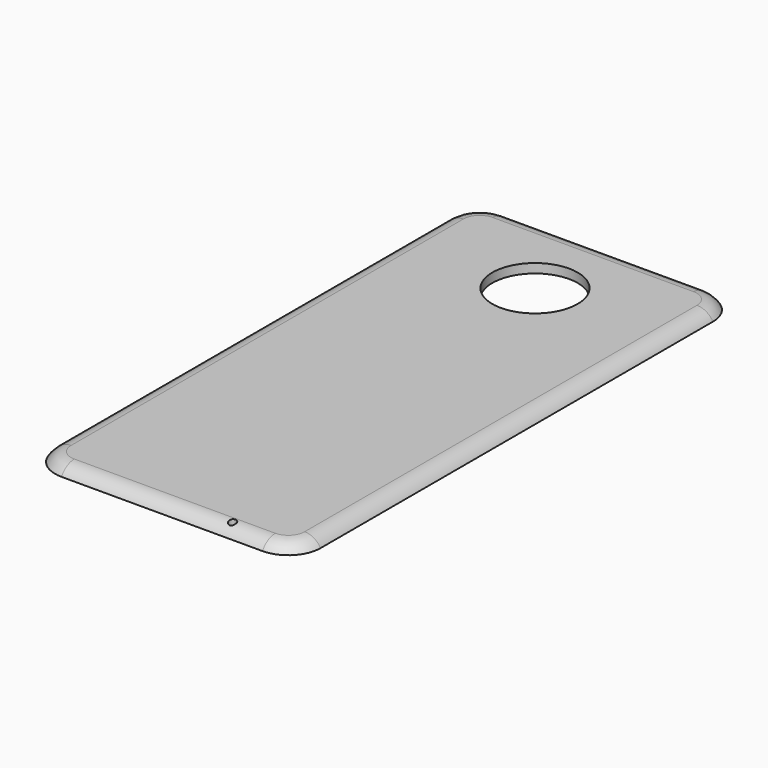
from build123d import *

# Parameters (mm, degrees)
F1_DEPTH     = 2.54
F2_R         = 11.75
F3_DEPTH     = 2.541
F4_R         = 8.89
F5_T1_DEPTH  = 135.128
F5_T3_DEPTH  = 55.372
F5_T6_ANGLE  = 90
F5_T8_ANGLE  = 90
F5_T10_ANGLE = 90
F5_T12_ANGLE = 90
F6_R         = 1
F7_DEPTH     = 2.541
F9_R         = 1.6
F8_R         = 1.6
F10_DEPTH    = 1.2
F11_R        = 2.794
F12_DEPTH    = 1.27


# Not quite as in the source:
# - a fillet or chamfer that OpenCascade refuses, or shapes differently, is made with other operations: its cross-section is extruded or revolved along the edge and cut away or added


with BuildPart() as f1:
    # F0 (on Top) → F1 (new body)
    with BuildSketch(Plane.XY):
        Polygon((36.576, 76.454), (0, 76.454), (-36.576, 76.454), (-36.576, 0), (-36.576, -76.454), (0, -76.454), (36.576, -76.454), (36.576, 0), align=None)
    extrude(amount=F1_DEPTH)

    # F2 (on face) → F3 (cut, through all)
    with BuildSketch(Plane.XY.offset(2.54)):
        with Locations((0, 52.004)):
            Circle(F2_R)
    extrude(amount=-F3_DEPTH, mode=Mode.SUBTRACT)

    # F4
    f4_edges = [f1.edges().sort_by_distance(p)[0] for p in [
        (-36.576, 76.454, 1.27),
        (36.576, 76.454, 1.27),
        (36.576, -76.454, 1.27),
        (-36.576, -76.454, 1.27),
    ]]
    fillet(f4_edges, radius=F4_R)

    # F5: fillet of radius 5.08 on 1 edges, made by hand

    # F5_s2 → F5_t1 (cut)
    with BuildSketch(Plane.XZ.offset(-67.564)):
        with BuildLine():
            ThreePointArc((32.1765909488, 2.54), (34.7165909488, 1.8594090512), (36.576, 0))
            Line((36.576, 0), (36.576, 2.54))
            Line((36.576, 2.54), (32.1765909488, 2.54))
        make_face()
        with BuildLine():
            ThreePointArc((-32.1765909488, 2.54), (-34.7165909488, 1.8594090512), (-36.576, 0))
            Line((-36.576, 0), (-36.576, 2.54))
            Line((-36.576, 2.54), (-32.1765909488, 2.54))
        make_face()
    extrude(amount=F5_T1_DEPTH, mode=Mode.SUBTRACT)

    # F5_s4 → F5_t3 (cut)
    with BuildSketch(Plane.YZ.offset(-27.686)):
        with BuildLine():
            ThreePointArc((-72.0545909488, 2.54), (-74.5945909488, 1.8594090512), (-76.454, 0))
            Line((-76.454, 0), (-76.454, 2.54))
            Line((-76.454, 2.54), (-72.0545909488, 2.54))
        make_face()
        with BuildLine():
            ThreePointArc((76.454, 0), (74.5945909488, 1.8594090512), (72.0545909488, 2.54))
            Line((72.0545909488, 2.54), (76.454, 2.54))
            Line((76.454, 2.54), (76.454, 0))
        make_face()
    extrude(amount=F5_T3_DEPTH, mode=Mode.SUBTRACT)

    # F5_s5 → F5_t6 (revolve, cut)
    with BuildSketch(Plane.YZ.offset(27.686)):
        with BuildLine():
            ThreePointArc((72.0545909488, 2.54), (74.5945909488, 1.8594090512), (76.454, 0))
            Line((76.454, 0), (76.454, 2.54))
            Line((76.454, 2.54), (72.0545909488, 2.54))
        make_face()
    revolve(axis=Axis((27.686, 67.564, 2.54), (0, 0, -1)), revolution_arc=F5_T6_ANGLE, mode=Mode.SUBTRACT)

    # F5_s7 → F5_t8 (revolve, cut)
    with BuildSketch(Plane.XZ.offset(67.564)):
        with BuildLine():
            ThreePointArc((32.1765909488, 2.54), (34.7165909488, 1.8594090512), (36.576, 0))
            Line((36.576, 0), (36.576, 2.54))
            Line((36.576, 2.54), (32.1765909488, 2.54))
        make_face()
    revolve(axis=Axis((27.686, -67.564, 2.54), (0, 0, -1)), revolution_arc=F5_T8_ANGLE, mode=Mode.SUBTRACT)

    # F5_s9 → F5_t10 (revolve, cut)
    with BuildSketch(Plane.XZ.offset(67.564)):
        with BuildLine():
            ThreePointArc((-32.1765909488, 2.54), (-34.7165909488, 1.8594090512), (-36.576, 0))
            Line((-36.576, 0), (-36.576, 2.54))
            Line((-36.576, 2.54), (-32.1765909488, 2.54))
        make_face()
    revolve(axis=Axis((-27.686, -67.564, 2.54), (0, 0, 1)), revolution_arc=F5_T10_ANGLE, mode=Mode.SUBTRACT)

    # F5_s11 → F5_t12 (revolve, cut)
    with BuildSketch(Plane.YZ.offset(-27.686)):
        with BuildLine():
            ThreePointArc((72.0545909488, 2.54), (74.5945909488, 1.8594090512), (76.454, 0))
            Line((76.454, 0), (76.454, 2.54))
            Line((76.454, 2.54), (72.0545909488, 2.54))
        make_face()
    revolve(axis=Axis((-27.686, 67.564, 2.54), (0, 0, 1)), revolution_arc=F5_T12_ANGLE, mode=Mode.SUBTRACT)

    # F6 (on face) → F7 (cut, through all)
    with BuildSketch(Plane(origin=(0, 0, 0), x_dir=(1, 0, 0), z_dir=(0, 0, -1))):
        with Locations((17.018, 73.406)):
            Circle(F6_R)
    extrude(amount=-F7_DEPTH, mode=Mode.SUBTRACT)

    # F9 (on face) + F8 (on face) → F10 (cut)
    with BuildSketch(Plane(origin=(0, 0, 0), x_dir=(1, 0, 0), z_dir=(0, 0, -1))):
        with Locations((19.736, 59.614)):
            Circle(F9_R)
        with Locations((-19.736, 59.614)):
            Circle(F9_R)
    with BuildSketch(Plane(origin=(0, 0, 0), x_dir=(1, 0, 0), z_dir=(0, 0, -1))):
        with Locations((-22.276, -62.154)):
            Circle(F8_R)
        with Locations((22.276, -62.154)):
            Circle(F8_R)
    extrude(amount=-F10_DEPTH, mode=Mode.SUBTRACT)

    # F11 (on face) → F12 (cut)
    with BuildSketch(Plane(origin=(0, 0, 0), x_dir=(1, 0, 0), z_dir=(0, 0, -1))):
        with Locations((0, 61.214)):
            Circle(F11_R)
    extrude(amount=-F12_DEPTH, mode=Mode.SUBTRACT)


solid = f1.part
